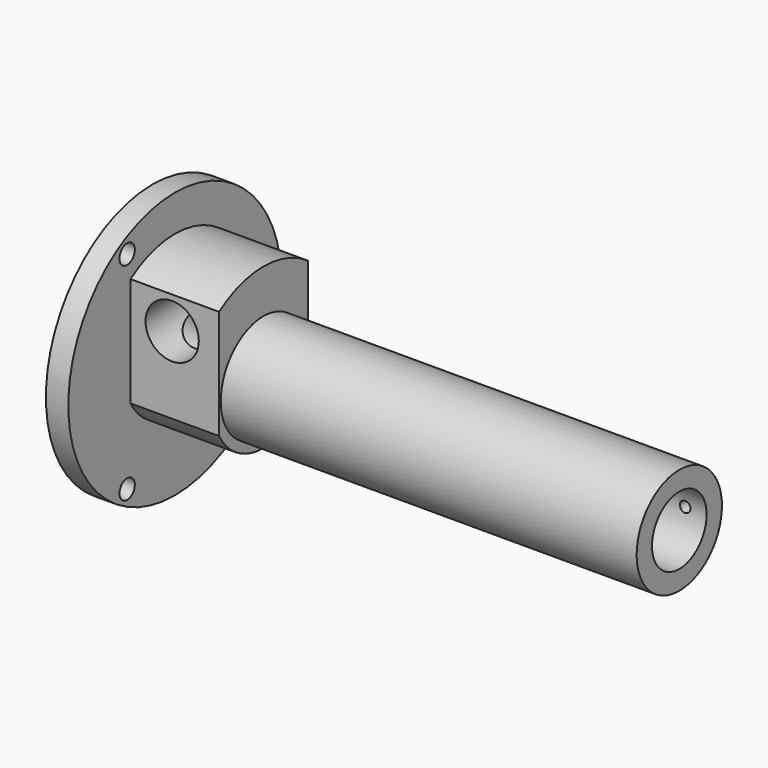
from build123d import *

# Parameters (mm, degrees)
F2_R      = 25
F3_DEPTH  = 41.5
F4_R      = 12.5
F5_DEPTH  = 30
F6_R      = 2.5
F7_DEPTH  = 62.501
F8_R      = 4.5
F9_DEPTH  = 13.5010001
F12_DEPTH = 14


with BuildPart() as f1:
    # F0 (on Front) → F1 (revolve)
    with BuildSketch(Plane.XZ):
        Polygon((10.5, 62.5), (0, 62.5), (0, 35), (-3, 35), (-3, 16), (247, 16), (247, 25), (10.5, 25), align=None)
    revolve(axis=Axis((-11.2489545718, 0, 0), (-1, 0, 0)))

    # F2 (on face) → F3 (join)
    with BuildSketch(Plane.YZ.offset(10.5)):
        with BuildLine():
            Line((26, -13.9373598648), (26, 37.3396572025))
            ThreePointArc((26, 37.3396572025), (0, 45.5), (-26, 37.3396572025))
            Line((-26, 37.3396572025), (-26, -13.9373598648))
            ThreePointArc((-26, -13.9373598648), (0, -29.5), (26, -13.9373598648))
        make_face()
        Circle(F2_R, mode=Mode.SUBTRACT)
    extrude(amount=F3_DEPTH)

    # F4 (on Front) → F5 (cut, symmetric)
    with BuildSketch(Plane.XZ):
        with Locations((30, 22.2058613113)):
            Circle(F4_R)
    extrude(amount=F5_DEPTH, both=True, mode=Mode.SUBTRACT)

    # F6 (on Front) → F7 (cut, through all)
    with BuildSketch(Plane.XZ):
        with Locations((237, 0)):
            Circle(F6_R)
    extrude(amount=-F7_DEPTH, mode=Mode.SUBTRACT)

    # F8 (on face) → F9 (cut, through all)
    with BuildSketch(Plane.YZ.offset(10.5)):
        with Locations((-28, 48.4974226119)):
            Circle(F8_R)
        with Locations((56, 0)):
            Circle(F8_R)
        with Locations((-28, -48.4974226119)):
            Circle(F8_R)
    extrude(amount=-F9_DEPTH, mode=Mode.SUBTRACT)

    # F11 (on offset) → F12 (join)
    with BuildSketch(Plane(origin=(24, 0, 0), x_dir=(0, -1, 0), z_dir=(-1, 0, 0))):
        with BuildLine():
            Line((-13, 2.5), (-15.8034806293, 2.5))
            ThreePointArc((-15.8034806293, 2.5), (-16, 0), (-15.8034806293, -2.5))
            Line((-15.8034806293, -2.5), (-13, -2.5))
            Line((-13, -2.5), (-13, 2.5))
        make_face()
        with BuildLine():
            ThreePointArc((15.8034806293, -2.5), (16, 0), (15.8034806293, 2.5))
            Line((15.8034806293, 2.5), (13, 2.5))
            Line((13, 2.5), (13, -2.5))
            Line((13, -2.5), (15.8034806293, -2.5))
        make_face()
    extrude(amount=-F12_DEPTH)


solid = f1.part
